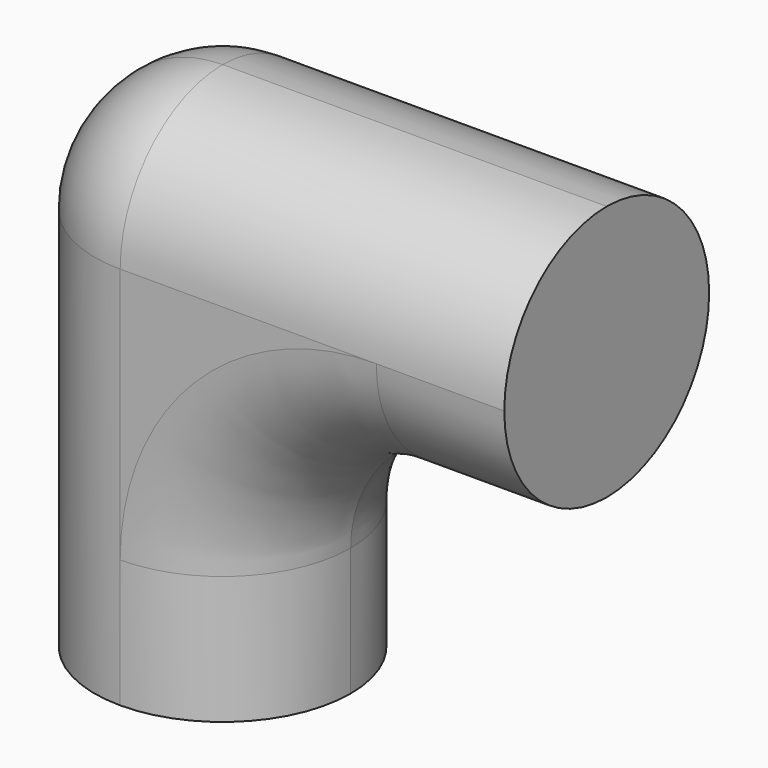
from build123d import *

# Parameters (mm, degrees)
F0_W     = 25.4
F0_H     = 25.4
F1_DEPTH = 25.4
F2_R     = 12.69999


# Not quite as in the source:
# - a fillet or chamfer is up to 0.001 mm smaller than in the source, because OpenCascade refuses the exact size


with BuildPart() as f1:
    # F0 (on Front) → F1 (new body)
    with BuildSketch(Plane.XZ):
        Polygon((-30.9433350532, 41.3746904978), (-56.3433350532, 41.3746904978), (-56.3433350532, -9.4253095022), (-30.9433350532, -9.4253095022), (-30.9433350532, 15.9746904978), align=None)
        with Locations((-18.2433350532, 28.6746904978)):
            Rectangle(F0_W, F0_H)
    extrude(amount=F1_DEPTH)

    # F2 (radius 12.7 in the source; OpenCascade refuses exactly that, so slightly less here)
    f2_edges = [f1.edges().sort_by_distance(p)[0] for p in [
        (-56.343335, 0, 15.97469),
        (-56.343335, -25.4, 15.97469),
        (-30.943335, -25.4, 41.37469),
        (-56.343335, -12.7, 41.37469),
        (-30.943335, 0, 41.37469),
        (-18.243335, -25.4, 15.97469),
        (-30.943335, -25.4, 3.27469),
        (-30.943335, 0, 3.27469),
        (-18.243335, 0, 15.97469),
        (-30.943335, -12.7, 15.97469),
    ]]
    fillet(f2_edges, radius=F2_R)


solid = f1.part
